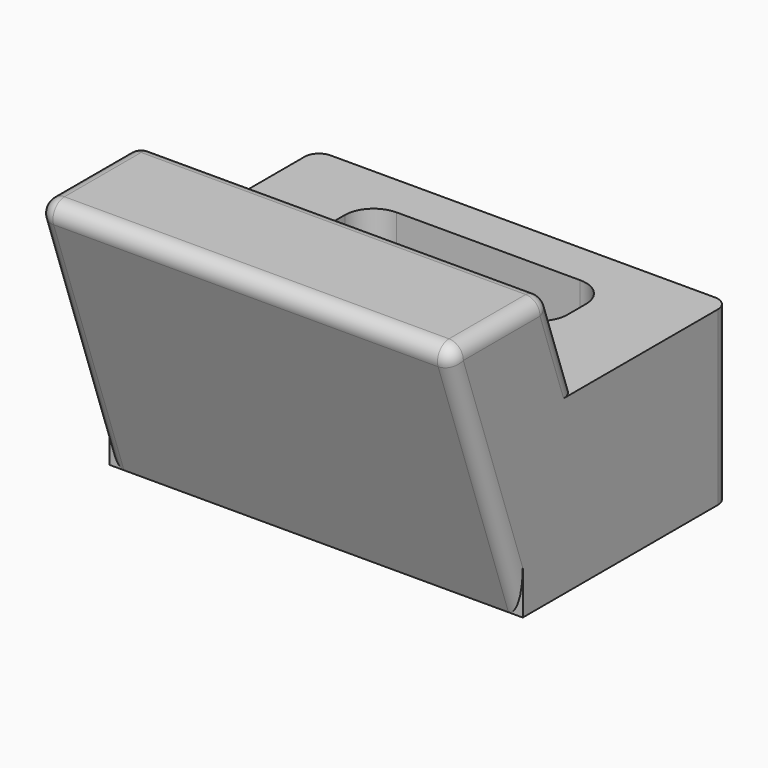
from build123d import *

# Parameters (mm, degrees)
F1_DEPTH = 6
F2_W     = 14.4
F2_H     = 4.4
F5_W     = 13.4
F5_H     = 3.4
F9_DEPTH = 4
F10_R    = 0.5


with BuildPart() as f1:
    # F0 (on Top) → F1 (new body)
    with BuildSketch(Plane.XY):
        Polygon((0, 2.8761399509), (0.5, 2.8761399509), (13.9, 2.8761399509), (14.4, 2.8761399509), (14.4, 3.3761399509), (0, 3.3761399509), align=None)
        Polygon((0, 10.3761399509), (0, 3.3761399509), (14.4, 3.3761399509), (14.4, 10.3761399509), (14.4, 11.8761399509), (12.9, 11.8761399509), (1.5, 11.8761399509), (0, 11.8761399509), align=None)
        with BuildLine():
            ThreePointArc((3, 9.3761399509), (3.2928932188, 10.0832467321), (4, 10.3761399509))
            Line((4, 10.3761399509), (10.4, 10.3761399509))
            ThreePointArc((10.4, 10.3761399509), (11.1071067812, 10.0832467321), (11.4, 9.3761399509))
            Line((11.4, 9.3761399509), (11.4, 8.5761399509))
            ThreePointArc((11.4, 8.5761399509), (11.1071067812, 7.8690331698), (10.4, 7.5761399509))
            Line((10.4, 7.5761399509), (4, 7.5761399509))
            ThreePointArc((4, 7.5761399509), (3.2928932188, 7.8690331698), (3, 8.5761399509))
            Line((3, 8.5761399509), (3, 9.3761399509))
        make_face(mode=Mode.SUBTRACT)
    extrude(amount=F1_DEPTH)

    # F4: sweep along a path in F3
    with BuildLine(Plane(origin=(0, 0, 0), x_dir=(0, -1, 0), z_dir=(-1, 0, 0))) as f4_path:
        Line((-2.8761399509, 0), (0.418709749, 9.4416082028))
    # F2 (on face) → F4 (sweep)
    with BuildSketch(Plane(origin=(0, 0, 0), x_dir=(1, 0, 0), z_dir=(0, 0, -1))):
        with Locations((7.2, -5.0770884661)):
            Rectangle(F2_W, F2_H)
    sweep(path=f4_path.line)

    # F7: sweep along a path in F6
    with BuildLine(Plane.YZ) as f7_path:
        Line((3.6174104522, 8.9695277927), (6.7475176671, 0))
    # F5 (on face) → F7 (sweep, cut)
    with BuildSketch(Plane(origin=(0, 0, 0), x_dir=(1, 0, 0), z_dir=(0, 0, -1))):
        with Locations((7.2, -5.0761399509)):
            Rectangle(F5_W, F5_H)
    sweep(path=f7_path.line, mode=Mode.SUBTRACT)

    # F8 (on Top) → F9 (cut)
    with BuildSketch(Plane.XY):
        Polygon((13.9, 11.3761399509), (12.4, 11.3761399509), (2, 11.3761399509), (0.5, 11.3761399509), (0.5, 9.8761399509), (0.5, 4.8761399509), (0.5, 3.3786750864), (2, 3.3761399509), (12.4, 3.3761399509), (13.9, 3.3761399509), (13.9, 4.8761399509), (13.9, 9.8761399509), align=None)
    extrude(amount=F9_DEPTH, mode=Mode.SUBTRACT)

    # F10
    f10_edges = [f1.edges().sort_by_distance(p)[0] for p in [
        (0, 1.782239, 9.441608),
        (7.2, 3.982239, 9.441608),
        (14.4, 1.782239, 9.441608),
        (7.2, -0.417761, 9.441608),
        (14.4, 11.87614, 3),
        (0, 11.87614, 3),
        (0.5, 11.37614, 2),
        (13.9, 11.37614, 2),
        (0.5, 1.811086, 4.484764),
        (13.9, 1.811086, 4.484764),
        (0, 4.58275, 7.720804),
        (0, 1.229189, 4.722163),
        (14.4, 4.58275, 7.720804),
        (0.5, 1.946033, 8.969528),
        (7.2, 0.246033, 8.969528),
        (7.2, 3.646033, 8.969528),
        (13.9, 1.946033, 8.969528),
        (14.4, 1.229189, 4.722163),
    ]]
    fillet(f10_edges, radius=F10_R)


solid = f1.part
